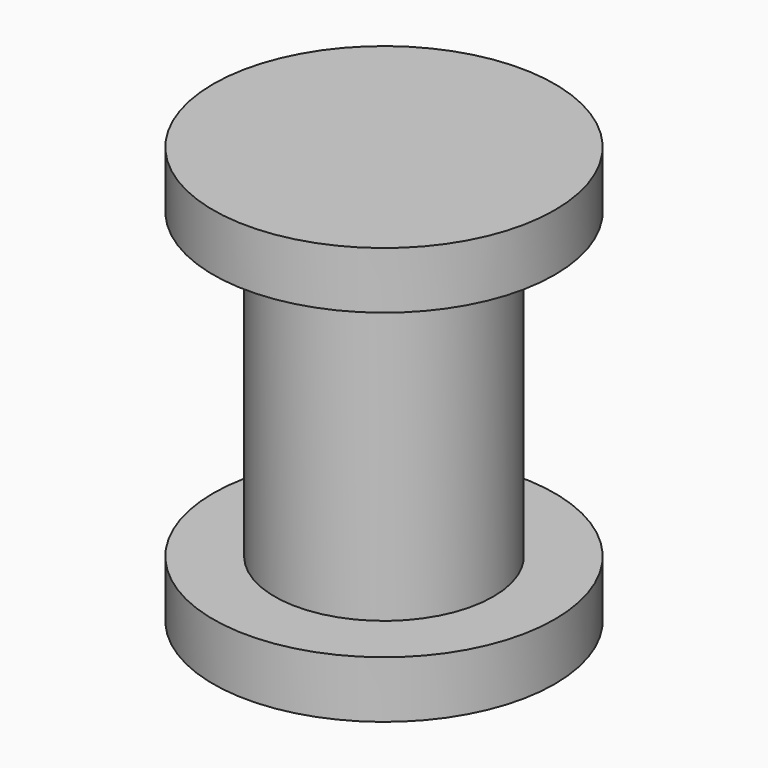
from build123d import *

# Parameters (mm, degrees)
F0_R     = 6.096
F1_DEPTH = 16.9164
F2_R     = 9.525
F2_R_2   = 6.096
F3_DEPTH = 3.175
F4_R     = 9.525
F5_DEPTH = 3.175


# Not quite as in the source:
# - a feature names something its author has since deleted; it is built from what else it names


with BuildPart() as f1:
    # F0 (on Top) → F1 (new body)
    with BuildSketch(Plane.XY):
        Circle(F0_R)
    extrude(amount=F1_DEPTH)

    # F2 (on face) → F3 (join)
    with BuildSketch(Plane.XY.offset(16.9164)):
        Circle(F2_R)
        Circle(F2_R_2, mode=Mode.SUBTRACT)
        Circle(F2_R_2)
    extrude(amount=F3_DEPTH)

    # F4 (on face) → F5 (join)
    with BuildSketch(Plane(origin=(0, 0, 0), x_dir=(1, 0, 0), z_dir=(0, 0, -1))):
        Circle(F4_R)
    extrude(amount=F5_DEPTH)


solid = f1.part
